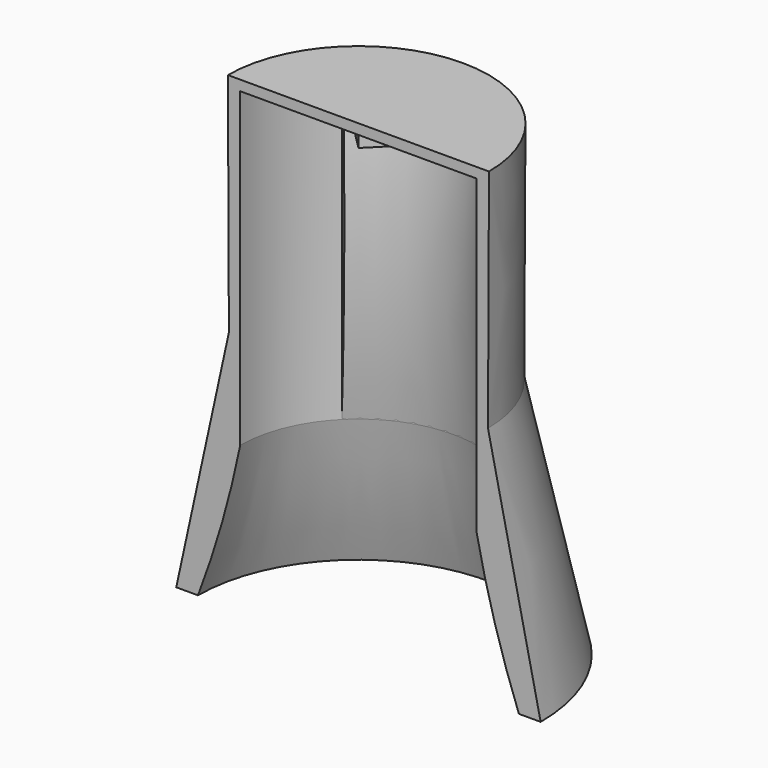
from build123d import *

# Parameters (mm, degrees)
F1_ANGLE       = 180
F2_ANGLE_START = 45
F2_ANGLE       = 90


# Not quite as in the source:
# - a feature names something its author has since deleted; it is built from what else it names


with BuildPart() as f1:
    # F0 (on Front) → F1 (revolve)
    with BuildSketch(Plane.XZ):
        with BuildLine():
            Line((0, 8.2611693069), (0, 9.2163154948))
            Line((0, 9.2163154948), (-5.092757754, 9.2163154948))
            Line((-5.092757754, 9.2163154948), (-12.192, 9.2163154948))
            Line((-12.192, 9.2163154948), (-12.0995361358, -11.9232786819))
            Line((-12.0995361358, -11.9232786819), (-17.018, -34.4716845052))
            Line((-17.018, -34.4716845052), (-14.986, -34.4716845052))
            ThreePointArc((-14.986, -34.4716845052), (-12.733545301, -27.7391345646), (-11.0408142209, -20.8445394087))
            Line((-11.0408142209, -20.8445394087), (-11.0408142209, 7.1843154948))
            Line((-11.0408142209, 7.1843154948), (-11.0408142209, 8.2611693069))
            Line((-11.0408142209, 8.2611693069), (0, 8.2611693069))
        make_face()
    revolve(axis=Axis((0, 0, 8.2003154948), (0, 0, -1)), revolution_arc=F1_ANGLE)


with BuildPart() as f2:
    # F0 (on Front) → F2 (revolve)
    with BuildSketch(Plane.XZ, mode=Mode.PRIVATE) as f2_sk:
        with BuildLine():
            Line((0, 7.1843154948), (0, 8.2611693069))
            Line((0, 8.2611693069), (-11.0408142209, 8.2611693069))
            Line((-11.0408142209, 8.2611693069), (-11.0408142209, 7.1843154948))
            Line((-11.0408142209, 7.1843154948), (-11.0408142209, -20.8445394087))
            ThreePointArc((-11.0408142209, -20.8445394087), (-9.3805061549, -6.8722716562), (-10.0076, 7.1843154948))
            Line((-10.0076, 7.1843154948), (0, 7.1843154948))
        make_face()
    revolve(f2_sk.sketch.rotate(Axis((0, 0, 8.2003154948), (0, 0, -1)), F2_ANGLE_START), axis=Axis((0, 0, 8.2003154948), (0, 0, -1)), revolution_arc=F2_ANGLE)


solid = Compound([f1.part, f2.part])
